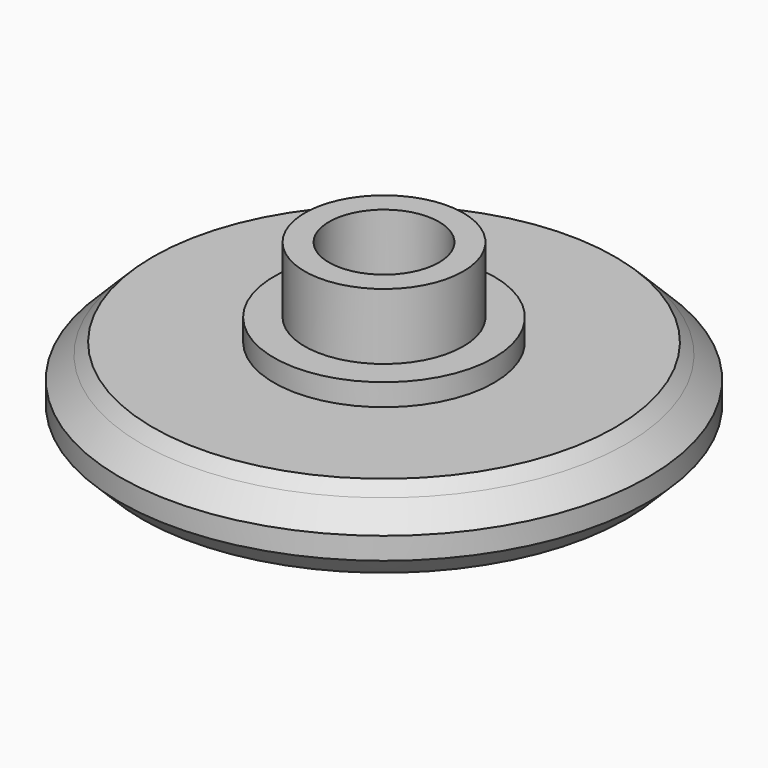
from build123d import *

# Parameters (mm, degrees)
F0_R      = 12
F0_R_2    = 11
F0_R_3    = 5
F0_R_4    = 4.1
F0_R_5    = 3
F1_DEPTH  = 2
F2_DEPTH  = 3.5
F3_SIZE   = 0.99999
F4_DEPTH  = 4.5
F5_DEPTH  = 7.5
F6_SIZE   = 1
F7_SIZE   = 0.5
F8_R      = 3
F8_R_2    = 2.5
F9_DEPTH  = 3
F10_R     = 4.1
F10_R_2   = 3.6
F11_DEPTH = 3


# Not quite as in the source:
# - a fillet or chamfer is up to 0.001 mm smaller than in the source, because OpenCascade refuses the exact size


with BuildPart() as f1:
    # F0 (on Top) → F1 (new body)
    with BuildSketch(Plane.XY):
        Circle(F0_R)
        Circle(F0_R_2, mode=Mode.SUBTRACT)
        Circle(F0_R_2)
        Circle(F0_R_3, mode=Mode.SUBTRACT)
        Circle(F0_R_3)
        Circle(F0_R_4, mode=Mode.SUBTRACT)
        Circle(F0_R_4)
        Circle(F0_R_5, mode=Mode.SUBTRACT)
        Circle(F0_R_5)
    extrude(amount=F1_DEPTH)

    # F0 (on Top) → F2 (join)
    with BuildSketch(Plane.XY):
        Circle(F0_R_2)
        Circle(F0_R_3, mode=Mode.SUBTRACT)
        Circle(F0_R_3)
        Circle(F0_R_4, mode=Mode.SUBTRACT)
        Circle(F0_R_4)
        Circle(F0_R_5, mode=Mode.SUBTRACT)
        Circle(F0_R_5)
    extrude(amount=F2_DEPTH)

    # F3 (size 1 in the source; OpenCascade refuses exactly that, so slightly less here)
    f3_edges = [f1.edges().sort_by_distance(p)[0] for p in [
        (-11, 0, 2),
    ]]
    chamfer(f3_edges, length=F3_SIZE)

    # F0 (on Top) → F4 (join)
    with BuildSketch(Plane.XY):
        Circle(F0_R_3)
        Circle(F0_R_4, mode=Mode.SUBTRACT)
        Circle(F0_R_4)
        Circle(F0_R_5, mode=Mode.SUBTRACT)
        Circle(F0_R_5)
    extrude(amount=F4_DEPTH)

    # F0 (on Top) → F5 (join)
    with BuildSketch(Plane.XY):
        Circle(F0_R_4)
        Circle(F0_R_5, mode=Mode.SUBTRACT)
    extrude(amount=F5_DEPTH)

    # F6
    f6_edges = [f1.edges().sort_by_distance(p)[0] for p in [
        (-12, 0, 0),
    ]]
    chamfer(f6_edges, length=F6_SIZE)

    # F7
    f7_edges = [f1.edges().sort_by_distance(p)[0] for p in [
        (-11, 0, 3.5),
    ]]
    chamfer(f7_edges, length=F7_SIZE)

    # F8 (on face) → F9 (join, through all)
    with BuildSketch(Plane.XY.offset(4.5)):
        Circle(F8_R)
        Circle(F8_R_2, mode=Mode.SUBTRACT)
    extrude(amount=F9_DEPTH)

    # F10 (on face) → F11 (cut, through all)
    with BuildSketch(Plane.XY.offset(7.5)):
        Circle(F10_R)
        Circle(F10_R_2, mode=Mode.SUBTRACT)
    extrude(amount=-F11_DEPTH, mode=Mode.SUBTRACT)


solid = f1.part
